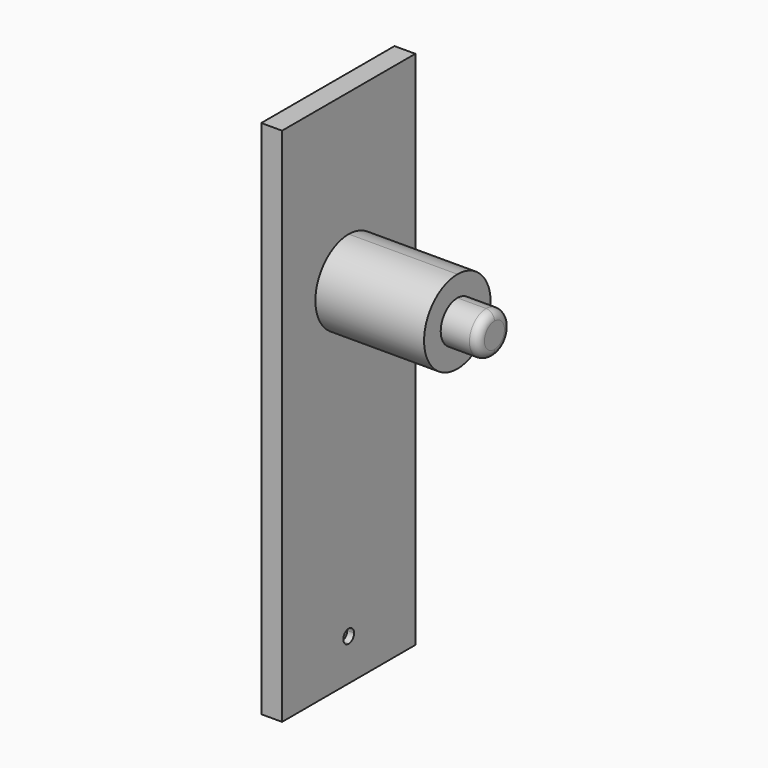
from build123d import *

# Parameters (mm, degrees)
F1_DEPTH = 6.35
F2_DEPTH = 39.497
F3_DEPTH = 50.8
F4_R     = 2.54
F6_DEPTH = 31.75


# Not quite as in the source:
# - a fillet or chamfer that OpenCascade refuses, or shapes differently, is made with other operations: its cross-section is extruded or revolved along the edge and cut away or added


with BuildPart() as f1:
    # F0 (on Right) → F1 (new body)
    with BuildSketch(Plane.YZ):
        with BuildLine():
            Line((0, 79.1307692308), (-25.4, 79.1307692308))
            Line((-25.4, 79.1307692308), (-25.4, -79.6192307692))
            Line((-25.4, -79.6192307692), (0, -79.6192307692))
            Line((0, -79.6192307692), (0, -68.9766307692))
            ThreePointArc((0, -68.9766307692), (-2.0574, -66.9192307692), (0, -64.8618307692))
            Line((0, -64.8618307692), (0, -54.2192307692))
            Line((0, -54.2192307692), (0, -41.5192307692))
            Line((0, -41.5192307692), (0, 15.6307692308))
            ThreePointArc((0, 15.6307692308), (-12.7, 28.3307692308), (0, 41.0307692308))
            Line((0, 41.0307692308), (0, 79.1307692308))
        make_face()
        with BuildLine():
            Line((25.4, 79.1307692308), (0, 79.1307692308))
            Line((0, 79.1307692308), (0, 41.0307692308))
            ThreePointArc((0, 41.0307692308), (8.9802561211, 37.3110253518), (12.7, 28.3307692308))
            ThreePointArc((12.7, 28.3307692308), (8.9802561211, 19.3505131097), (0, 15.6307692308))
            Line((0, 15.6307692308), (0, -41.5192307692))
            Line((0, -41.5192307692), (0, -54.2192307692))
            Line((0, -54.2192307692), (0, -64.8618307692))
            ThreePointArc((0, -64.8618307692), (1.4548014916, -65.4644292776), (2.0574, -66.9192307692))
            ThreePointArc((2.0574, -66.9192307692), (1.4548014916, -68.3740322608), (0, -68.9766307692))
            Line((0, -68.9766307692), (0, -79.6192307692))
            Line((0, -79.6192307692), (25.4, -79.6192307692))
            Line((25.4, -79.6192307692), (25.4, 79.1307692308))
        make_face()
    extrude(amount=F1_DEPTH)

    # F0 (on Right) → F2 (join)
    with BuildSketch(Plane.YZ):
        with BuildLine():
            Line((0, 37.8557692308), (0, 41.0307692308))
            ThreePointArc((0, 41.0307692308), (-12.7, 28.3307692308), (0, 15.6307692308))
            Line((0, 15.6307692308), (0, 18.8057692308))
            ThreePointArc((0, 18.8057692308), (-9.525, 28.3307692308), (0, 37.8557692308))
        make_face()
        with BuildLine():
            ThreePointArc((12.7, 28.3307692308), (8.9802561211, 37.3110253518), (0, 41.0307692308))
            Line((0, 41.0307692308), (0, 37.8557692308))
            ThreePointArc((0, 37.8557692308), (6.7351920908, 35.0659613216), (9.525, 28.3307692308))
            ThreePointArc((9.525, 28.3307692308), (6.7351920908, 21.59557714), (0, 18.8057692308))
            Line((0, 18.8057692308), (0, 15.6307692308))
            ThreePointArc((0, 15.6307692308), (8.9802561211, 19.3505131097), (12.7, 28.3307692308))
        make_face()
        with BuildLine():
            Line((0, 34.6807692308), (0, 37.8557692308))
            ThreePointArc((0, 37.8557692308), (-9.525, 28.3307692308), (0, 18.8057692308))
            Line((0, 18.8057692308), (0, 21.9807692308))
            ThreePointArc((0, 21.9807692308), (-6.35, 28.3307692308), (0, 34.6807692308))
        make_face()
        with BuildLine():
            ThreePointArc((9.525, 28.3307692308), (6.7351920908, 35.0659613216), (0, 37.8557692308))
            Line((0, 37.8557692308), (0, 34.6807692308))
            ThreePointArc((0, 34.6807692308), (4.4901280605, 32.8208972913), (6.35, 28.3307692308))
            ThreePointArc((6.35, 28.3307692308), (4.4901280605, 23.8406411702), (0, 21.9807692308))
            Line((0, 21.9807692308), (0, 18.8057692308))
            ThreePointArc((0, 18.8057692308), (6.7351920908, 21.59557714), (9.525, 28.3307692308))
        make_face()
    extrude(amount=F2_DEPTH)

    # F0 (on Right) → F3 (join)
    with BuildSketch(Plane.YZ):
        with BuildLine():
            Line((0, 28.3307692308), (0, 34.6807692308))
            ThreePointArc((0, 34.6807692308), (-6.35, 28.3307692308), (0, 21.9807692308))
            Line((0, 21.9807692308), (0, 28.3307692308))
        make_face()
        with BuildLine():
            ThreePointArc((6.35, 28.3307692308), (4.4901280605, 32.8208972913), (0, 34.6807692308))
            Line((0, 34.6807692308), (0, 28.3307692308))
            Line((0, 28.3307692308), (0, 21.9807692308))
            ThreePointArc((0, 21.9807692308), (4.4901280605, 23.8406411702), (6.35, 28.3307692308))
        make_face()
    extrude(amount=F3_DEPTH)

    # F4
    f4_edges = [f1.edges().sort_by_distance(p)[0] for p in [
        (50.8, 0, 34.680769),
    ]]
    fillet(f4_edges, radius=F4_R)

    # F5: chamfer of 2.7178 x 4.2672 on 1 edges, made by hand

    # F5_s1 → F5_t2 (revolve, cut)
    with BuildSketch(Plane.XZ):
        Polygon((4.2672, -64.8618307692), (0, -62.1440307692), (0, -64.8618307692), align=None)
    revolve(axis=Axis((0, 0, -66.9192307692), (-1, 0, 0)), mode=Mode.SUBTRACT)

    # F0 (on Right) → F6 (cut)
    with BuildSketch(Plane.YZ):
        with BuildLine():
            Line((0, 34.6807692308), (0, 37.8557692308))
            ThreePointArc((0, 37.8557692308), (-9.525, 28.3307692308), (0, 18.8057692308))
            Line((0, 18.8057692308), (0, 21.9807692308))
            ThreePointArc((0, 21.9807692308), (-6.35, 28.3307692308), (0, 34.6807692308))
        make_face()
        with BuildLine():
            Line((0, 28.3307692308), (0, 34.6807692308))
            ThreePointArc((0, 34.6807692308), (-6.35, 28.3307692308), (0, 21.9807692308))
            Line((0, 21.9807692308), (0, 28.3307692308))
        make_face()
        with BuildLine():
            ThreePointArc((6.35, 28.3307692308), (4.4901280605, 32.8208972913), (0, 34.6807692308))
            Line((0, 34.6807692308), (0, 28.3307692308))
            Line((0, 28.3307692308), (0, 21.9807692308))
            ThreePointArc((0, 21.9807692308), (4.4901280605, 23.8406411702), (6.35, 28.3307692308))
        make_face()
        with BuildLine():
            ThreePointArc((9.525, 28.3307692308), (6.7351920908, 35.0659613216), (0, 37.8557692308))
            Line((0, 37.8557692308), (0, 34.6807692308))
            ThreePointArc((0, 34.6807692308), (4.4901280605, 32.8208972913), (6.35, 28.3307692308))
            ThreePointArc((6.35, 28.3307692308), (4.4901280605, 23.8406411702), (0, 21.9807692308))
            Line((0, 21.9807692308), (0, 18.8057692308))
            ThreePointArc((0, 18.8057692308), (6.7351920908, 21.59557714), (9.525, 28.3307692308))
        make_face()
    extrude(amount=F6_DEPTH, mode=Mode.SUBTRACT)


solid = f1.part
